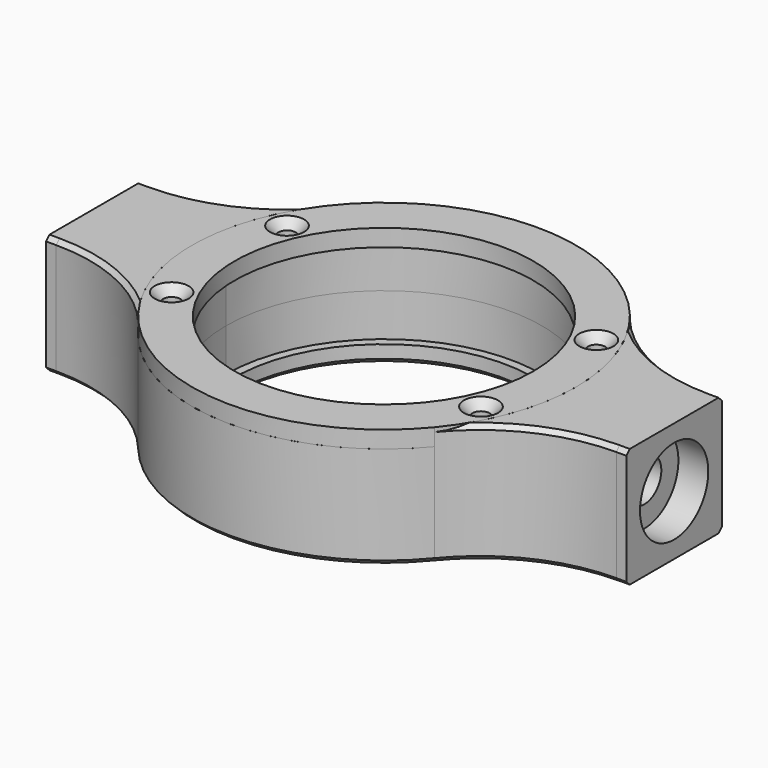
from build123d import *

# Parameters (mm, degrees)
F0_R          = 1
F0_R_2        = 18.5
F1_DEPTH      = 7
F1_DEPTH_BACK = 7
F2_START      = -5
F0_R_3        = 17.5
F2_DEPTH      = 2
F3_R          = 20
F4_R          = 1
F4_R_2        = 18.5
F5_DEPTH      = 2
F4_R_3        = 17.5
F6_DEPTH      = 2
F7_T1_DEPTH   = 2.4643546294
F7_T3_DEPTH   = 2.4643546294
F7_T6_ANGLE   = 61.6105922117
F7_T8_ANGLE   = 61.6105922117
F7_T10_ANGLE  = 61.6105922117
F7_T12_ANGLE  = 61.6105922117
F7_T14_ANGLE  = 50.5581979624
F7_T16_ANGLE  = 101.1163959248
F7_T22_ANGLE  = 50.5581979624
F7_T24_ANGLE  = 50.5581979624
F7_T26_ANGLE  = 101.1163959248
F7_T28_ANGLE  = 50.5581979624
F8_SIZE       = 1
F9_R          = 5
F9_R_2        = 2.5
F10_DEPTH     = 3.5
F11_DEPTH     = 15


# Not quite as in the source:
# - a fillet or chamfer that OpenCascade refuses, or shapes differently, is made with other operations: its cross-section is extruded or revolved along the edge and cut away or added


with BuildPart() as f1:
    # F0 (on Top) → F1 (new body, two sides)
    with BuildSketch(Plane.XY) as f1_sk:
        with BuildLine():
            Line((34, 7), (21.3834047803, 7))
            ThreePointArc((21.3834047803, 7), (0, 22.5), (-21.3834047803, 7))
            Line((-21.3834047803, 7), (-34, 7))
            Line((-34, 7), (-34, -7))
            Line((-34, -7), (-21.3834047803, -7))
            ThreePointArc((-21.3834047803, -7), (0, -22.5), (21.3834047803, -7))
            Line((21.3834047803, -7), (34, -7))
            Line((34, -7), (34, 7))
        make_face()
        with Locations((-18.1261557407, -8.4523652348)):
            Circle(F0_R, mode=Mode.SUBTRACT)
        with Locations((18.1261557407, -8.4523652348)):
            Circle(F0_R, mode=Mode.SUBTRACT)
        with Locations((-18.1261557407, 8.4523652348)):
            Circle(F0_R, mode=Mode.SUBTRACT)
        Circle(F0_R_2, mode=Mode.SUBTRACT)
        with Locations((18.1261557407, 8.4523652348)):
            Circle(F0_R, mode=Mode.SUBTRACT)
    extrude(amount=F1_DEPTH)
    extrude(f1_sk.sketch, amount=-F1_DEPTH_BACK)

    # F0 (on Top) → F2 (join)
    with BuildSketch(Plane.XY.offset(F2_START)):
        Circle(F0_R_2)
        Circle(F0_R_3, mode=Mode.SUBTRACT)
        with Locations((18.1261557407, 8.4523652348)):
            Circle(F0_R)
        with Locations((18.1261557407, -8.4523652348)):
            Circle(F0_R)
        with Locations((-18.1261557407, -8.4523652348)):
            Circle(F0_R)
        with Locations((-18.1261557407, 8.4523652348)):
            Circle(F0_R)
    extrude(amount=-F2_DEPTH)

    # F3
    f3_edges = [f1.edges().sort_by_distance(p)[0] for p in [
        (21.383405, 7, 0),
        (21.383405, -7, 0),
        (-21.383405, -7, 0),
        (-21.383405, 7, 0),
    ]]
    fillet(f3_edges, radius=F3_R)

    # F4 (on face) → F5 (cut)
    with BuildSketch(Plane.XY.offset(7)):
        with BuildLine():
            ThreePointArc((17.3760812812, -14.2941176471), (21.1803190348, -7.5923702219), (22.5, 0))
            ThreePointArc((22.5, 0), (21.1803190348, 7.5923702219), (17.3760812812, 14.2941176471))
            ThreePointArc((17.3760812812, 14.2941176471), (0, 22.5), (-17.3760812812, 14.2941176471))
            ThreePointArc((-17.3760812812, 14.2941176471), (-22.5, 0), (-17.3760812812, -14.2941176471))
            ThreePointArc((-17.3760812812, -14.2941176471), (0, -22.5), (17.3760812812, -14.2941176471))
        make_face()
        with Locations((-18.1261557407, -8.4523652348)):
            Circle(F4_R, mode=Mode.SUBTRACT)
        with Locations((18.1261557407, -8.4523652348)):
            Circle(F4_R, mode=Mode.SUBTRACT)
        with Locations((-18.1261557407, 8.4523652348)):
            Circle(F4_R, mode=Mode.SUBTRACT)
        Circle(F4_R_2, mode=Mode.SUBTRACT)
        with Locations((18.1261557407, 8.4523652348)):
            Circle(F4_R, mode=Mode.SUBTRACT)
        with Locations((18.1261557407, -8.4523652348)):
            Circle(F4_R)
        with Locations((18.1261557407, 8.4523652348)):
            Circle(F4_R)
        with Locations((-18.1261557407, 8.4523652348)):
            Circle(F4_R)
        with Locations((-18.1261557407, -8.4523652348)):
            Circle(F4_R)
    extrude(amount=-F5_DEPTH, mode=Mode.SUBTRACT)

    # F7: chamfer of 0.5 on 8 edges, made by hand

    # F7_s2 → F7_t1 (cut)
    with BuildSketch(Plane.YZ.offset(-35.285841494)):
        Polygon((6.5, -7), (7, -6.5), (7, -7), align=None)
        Polygon((-6.5, -7), (-7, -6.5), (-7, -7), align=None)
        Polygon((7, 6.5), (6.5, 7), (7, 7), align=None)
        Polygon((-7, 6.5), (-6.5, 7), (-7, 7), align=None)
    extrude(amount=F7_T1_DEPTH, mode=Mode.SUBTRACT)

    # F7_s4 → F7_t3 (cut)
    with BuildSketch(Plane.YZ.offset(32.8214868646)):
        Polygon((6.5, -7), (7, -6.5), (7, -7), align=None)
        Polygon((-7, -6.5), (-6.5, -7), (-7, -7), align=None)
        Polygon((6.5, 7), (7, 6.5), (7, 7), align=None)
        Polygon((-7, 6.5), (-6.5, 7), (-7, 7), align=None)
    extrude(amount=F7_T3_DEPTH, mode=Mode.SUBTRACT)

    # F7_s5 → F7_t6 (revolve, cut)
    with BuildSketch(Plane(origin=(3.873837059, -7.1676786017, 0), x_dir=(0, 0, 1), z_dir=(0.4754615812, -0.879736486, 0))):
        Polygon((6.5, 21.7117222121), (7, 21.2117222121), (7, 21.7117222121), align=None)
    revolve(axis=Axis((-32.8214868646, -27, 7), (0, 0, 1)), revolution_arc=F7_T6_ANGLE, mode=Mode.SUBTRACT)

    # F7_s7 → F7_t8 (revolve, cut)
    with BuildSketch(Plane(origin=(3.873837059, 7.1676786017, 0), x_dir=(0, 0, 1), z_dir=(0.4754615812, 0.879736486, 0))):
        Polygon((6.5, -21.7117222121), (7, -21.2117222121), (7, -21.7117222121), align=None)
    revolve(axis=Axis((-32.8214868646, 27, 7), (0, 0, -1)), revolution_arc=F7_T8_ANGLE, mode=Mode.SUBTRACT)

    # F7_s9 → F7_t10 (revolve, cut)
    with BuildSketch(Plane.YZ.offset(32.8214868646)):
        Polygon((-6.5, 7), (-7, 6.5), (-7, 7), align=None)
    revolve(axis=Axis((32.8214868646, -27, 7), (0, 0, 1)), revolution_arc=F7_T10_ANGLE, mode=Mode.SUBTRACT)

    # F7_s11 → F7_t12 (revolve, cut)
    with BuildSketch(Plane.YZ.offset(32.8214868646)):
        Polygon((6.5, 7), (7, 6.5), (7, 7), align=None)
    revolve(axis=Axis((32.8214868646, 27, 7), (0, 0, -1)), revolution_arc=F7_T12_ANGLE, mode=Mode.SUBTRACT)

    # F7_s13 → F7_t14 (revolve, cut)
    with BuildSketch(Plane.YZ.offset(32.8214868646)):
        Polygon((-7, -6.5), (-6.5, -7), (-7, -7), align=None)
    revolve(axis=Axis((32.8214868646, -27, -7), (0, 0, 1)), revolution_arc=F7_T14_ANGLE, mode=Mode.SUBTRACT)

    # F7_s15 → F7_t16 (revolve, cut)
    with BuildSketch(Plane(origin=(0, 0, 0), x_dir=(0, 0, 1), z_dir=(0.6352941176, -0.7722702792, 0))):
        Polygon((-7, -22), (-6.5, -22.5), (-7, -22.5), align=None)
    revolve(axis=Axis((0, 0, -7), (0, 0, 1)), revolution_arc=F7_T16_ANGLE, mode=Mode.SUBTRACT)

    # F7_s17 → F7_t18 (revolve, cut)
    with BuildSketch(Plane.XZ):
        Polygon((18, -7), (17.5, -6.5), (17.5, -7), align=None)
    revolve(axis=Axis((0, 0, -7), (0, 0, 1)), mode=Mode.SUBTRACT)

    # F7_s19 → F7_t20 (revolve, cut)
    with BuildSketch(Plane.XZ):
        Polygon((19, 5), (18.5, 4.5), (18.5, 5), align=None)
    revolve(axis=Axis((0, 0, 5), (0, 0, 1)), mode=Mode.SUBTRACT)

    # F7_s21 → F7_t22 (revolve, cut)
    with BuildSketch(Plane.YZ.offset(32.8214868646)):
        Polygon((6.5, -7), (7, -6.5), (7, -7), align=None)
    revolve(axis=Axis((32.8214868646, 27, -7), (0, 0, -1)), revolution_arc=F7_T22_ANGLE, mode=Mode.SUBTRACT)

    # F7_s23 → F7_t24 (revolve, cut)
    with BuildSketch(Plane(origin=(0, 0, 0), x_dir=(0, 0, 1), z_dir=(0.6352941176, 0.7722702792, 0))):
        Polygon((-7, -22), (-6.5, -22.5), (-7, -22.5), align=None)
    revolve(axis=Axis((-32.8214868646, 27, -7), (0, 0, -1)), revolution_arc=F7_T24_ANGLE, mode=Mode.SUBTRACT)

    # F7_s25 → F7_t26 (revolve, cut)
    with BuildSketch(Plane(origin=(0, 0, 0), x_dir=(0, 0, 1), z_dir=(-0.6352941176, 0.7722702792, 0))):
        Polygon((-7, -22), (-6.5, -22.5), (-7, -22.5), align=None)
    revolve(axis=Axis((0, 0, -7), (0, 0, 1)), revolution_arc=F7_T26_ANGLE, mode=Mode.SUBTRACT)

    # F7_s27 → F7_t28 (revolve, cut)
    with BuildSketch(Plane(origin=(0, 0, 0), x_dir=(0, 0, 1), z_dir=(0.6352941176, -0.7722702792, 0))):
        Polygon((-7, 22), (-6.5, 22.5), (-7, 22.5), align=None)
    revolve(axis=Axis((-32.8214868646, -27, -7), (0, 0, 1)), revolution_arc=F7_T28_ANGLE, mode=Mode.SUBTRACT)

    # F9 (on face) → F10 (cut)
    with BuildSketch(Plane(origin=(-34, 0, 0), x_dir=(0, -1, 0), z_dir=(-1, 0, 0))):
        Circle(F9_R)
        Circle(F9_R_2, mode=Mode.SUBTRACT)
        Circle(F9_R_2)
    extrude(amount=-F10_DEPTH, mode=Mode.SUBTRACT)

    # F9 (on face) → F11 (cut)
    with BuildSketch(Plane(origin=(-34, 0, 0), x_dir=(0, -1, 0), z_dir=(-1, 0, 0))):
        Circle(F9_R_2)
    extrude(amount=-F11_DEPTH, mode=Mode.SUBTRACT)

    # F12: F1 across plane


with BuildPart() as f6:
    # F4 (on face) → F6 (new body)
    with BuildSketch(Plane.XY.offset(7)):
        with BuildLine():
            ThreePointArc((17.3760812812, -14.2941176471), (21.1803190348, -7.5923702219), (22.5, 0))
            ThreePointArc((22.5, 0), (21.1803190348, 7.5923702219), (17.3760812812, 14.2941176471))
            ThreePointArc((17.3760812812, 14.2941176471), (0, 22.5), (-17.3760812812, 14.2941176471))
            ThreePointArc((-17.3760812812, 14.2941176471), (-22.5, 0), (-17.3760812812, -14.2941176471))
            ThreePointArc((-17.3760812812, -14.2941176471), (0, -22.5), (17.3760812812, -14.2941176471))
        make_face()
        with Locations((-18.1261557407, -8.4523652348)):
            Circle(F4_R, mode=Mode.SUBTRACT)
        with Locations((18.1261557407, -8.4523652348)):
            Circle(F4_R, mode=Mode.SUBTRACT)
        with Locations((-18.1261557407, 8.4523652348)):
            Circle(F4_R, mode=Mode.SUBTRACT)
        Circle(F4_R_2, mode=Mode.SUBTRACT)
        with Locations((18.1261557407, 8.4523652348)):
            Circle(F4_R, mode=Mode.SUBTRACT)
        Circle(F4_R_2)
        Circle(F4_R_3, mode=Mode.SUBTRACT)
    extrude(amount=-F6_DEPTH)

    # F8
    f8_edges = [f6.edges().sort_by_distance(p)[0] for p in [
        (17.126156, 8.452365, 7),
        (17.126156, -8.452365, 7),
        (-19.126156, -8.452365, 7),
        (-19.126156, 8.452365, 7),
    ]]
    chamfer(f8_edges, length=F8_SIZE)


with BuildPart() as f1_1:
    add(f1.part)
    add(f1.part.mirror(Plane.YZ), mode=Mode.INTERSECT)


solid = Compound([f6.part, f1_1.part])
